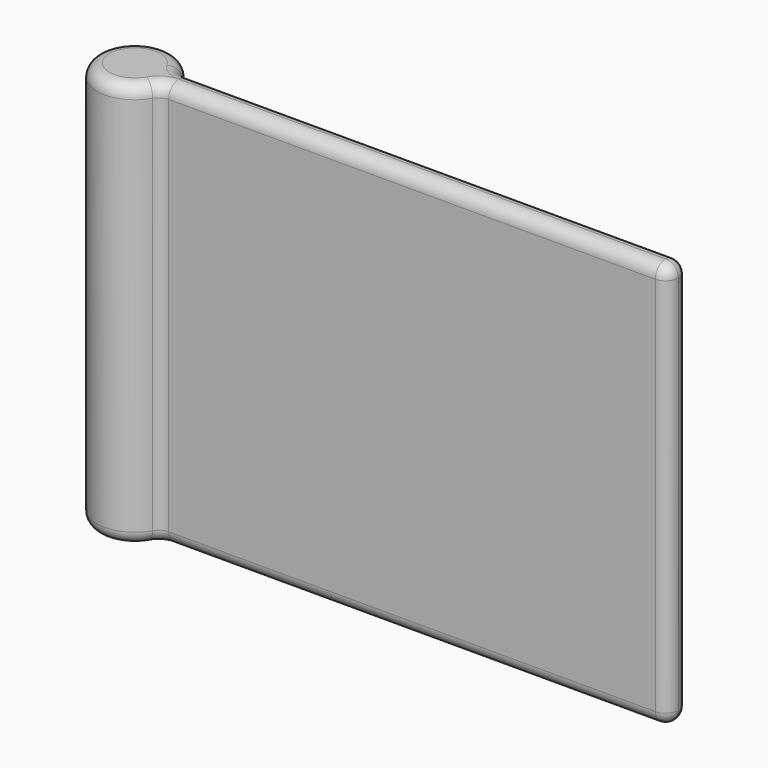
from build123d import *

# Parameters (mm, degrees)
F1_DEPTH = 25.4
F2_R     = 0.79374


# Not quite as in the source:
# - a fillet or chamfer is up to 0.001 mm smaller than in the source, because OpenCascade refuses the exact size
# - a feature names something its author has since deleted; it is built from what else it names


with BuildPart() as f1:
    # F0 (on Top) → F1 (new body)
    with BuildSketch(Plane.XY):
        with BuildLine():
            ThreePointArc((2.2450640303, -0.79375), (2.3469565702, -0.4026740868), (2.38125, 0))
            ThreePointArc((2.38125, 0), (2.3469565702, 0.4026740868), (2.2450640303, 0.79375))
            ThreePointArc((2.2450640303, 0.79375), (-2.38125, 0), (2.2450640303, -0.79375))
        make_face()
        with BuildLine():
            ThreePointArc((2.2450640303, 0.79375), (2.3469565702, 0.4026740868), (2.38125, 0))
            ThreePointArc((2.38125, 0), (2.3469565702, -0.4026740868), (2.2450640303, -0.79375))
            Line((2.2450640303, -0.79375), (33.9950640303, -0.79375))
            Line((33.9950640303, -0.79375), (33.9950640303, 0))
            Line((33.9950640303, 0), (33.9950640303, 0.79375))
            Line((33.9950640303, 0.79375), (2.2450640303, 0.79375))
        make_face()
    extrude(amount=F1_DEPTH)

    # F2 (radius 0.79375 in the source; OpenCascade refuses exactly that, so slightly less here)
    f2_edges = [f1.edges().sort_by_distance(p)[0] for p in [
        (-2.38125, 0, 25.4),
        (18.120064, -0.79375, 25.4),
        (33.995064, 0, 25.4),
        (18.120064, 0.79375, 25.4),
        (-2.38125, 0, 0),
        (18.120064, -0.79375, 0),
        (33.995064, 0, 0),
        (18.120064, 0.79375, 0),
        (33.995064, 0.79375, 12.7),
        (2.245064, 0.79375, 12.7),
        (2.245064, -0.79375, 12.7),
        (33.995064, -0.79375, 12.7),
    ]]
    fillet(f2_edges, radius=F2_R)


solid = f1.part
